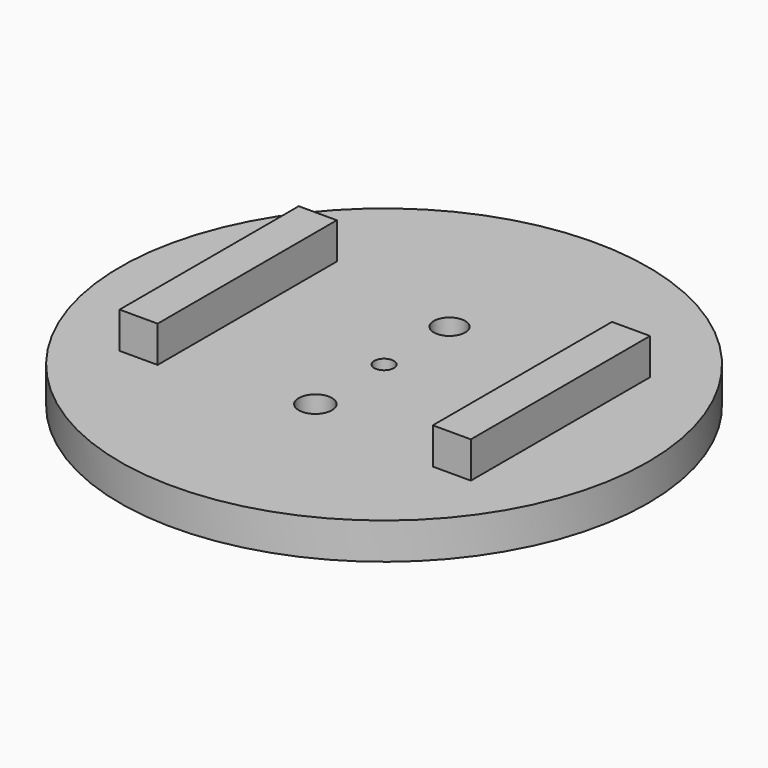
from build123d import *

# Parameters (mm, degrees)
F0_R     = 36.3144122586
F3_DEPTH = 5
F1_W     = 5.236171186
F1_H     = 30.8128492907
F4_DEPTH = 10
F2_R     = 2.2829264836
F2_R_2   = 1.3509728807
F2_R_3   = 2.1549795906
F5_DEPTH = 25
F7_DEPTH = 2


with BuildPart() as f3:
    # F0 (on Top) → F3 (new body)
    with BuildSketch(Plane.XY):
        Circle(F0_R)
    extrude(amount=F3_DEPTH)

    # F1 (on Top) → F4 (join)
    with BuildSketch(Plane.XY):
        with Locations((21.547390148, 0.1232274808)):
            Rectangle(F1_W, F1_H)
        Polygon((-24.165475741, 15.5296521261), (-24.165475741, 0), (-24.165475741, -15.2831971645), (-18.9293045551, -15.2831971645), (-18.9293045551, 15.5296521261), align=None)
    extrude(amount=F4_DEPTH)

    # F2 (on Top) → F5 (cut)
    with BuildSketch(Plane.XY):
        with Locations((0, -11.8196206167)):
            Circle(F2_R)
        Circle(F2_R_2)
        with Locations((0, 11.250000447)):
            Circle(F2_R_3)
    extrude(amount=F5_DEPTH, mode=Mode.SUBTRACT)

    # F6 (on Top) → F7 (cut)
    with BuildSketch(Plane.XY):
        with BuildLine():
            ThreePointArc((-0.3703859768, -3.5693595734), (2.402953818, -2.6652066495), (3.5885252592, 0))
            ThreePointArc((3.5885252592, 0), (2.402953818, 2.6652066495), (-0.3703859768, 3.5693595734))
            ThreePointArc((-0.3703859768, 3.5693595734), (-3.5885252592, 0), (-0.3703859768, -3.5693595734))
        make_face()
        with BuildLine():
            ThreePointArc((-0.3703859768, 3.5693595734), (2.402953818, 2.6652066495), (3.5885252592, 0))
            ThreePointArc((3.5885252592, 0), (2.402953818, -2.6652066495), (-0.3703859768, -3.5693595734))
            Line((-0.3703859768, -3.5693595734), (0, -3.6077938568))
            Line((0, -3.6077938568), (13.7103013694, -2.3183212426))
            ThreePointArc((13.7103013694, -2.3183212426), (11.3919801268, 0), (13.7103013694, 2.3183212426))
            Line((13.7103013694, 2.3183212426), (0, 3.6077938568))
            Line((0, 3.6077938568), (-0.3703859768, 3.5693595734))
        make_face()
        with BuildLine():
            ThreePointArc((-0.3703859768, -3.5693595734), (-3.5885252592, 0), (-0.3703859768, 3.5693595734))
            Line((-0.3703859768, 3.5693595734), (-12.5144906342, 2.3091877811))
            ThreePointArc((-12.5144906342, 2.3091877811), (-10.8816482952, 1.632842339), (-10.2053028531, 0))
            ThreePointArc((-10.2053028531, 0), (-10.8816482952, -1.632842339), (-12.5144906342, -2.3091877811))
            Line((-12.5144906342, -2.3091877811), (-0.3703859768, -3.5693595734))
        make_face()
        with BuildLine():
            Line((-12.5144906342, 0), (-12.5144906342, 2.3091877811))
            ThreePointArc((-12.5144906342, 2.3091877811), (-14.8236784153, 0), (-12.5144906342, -2.3091877811))
            Line((-12.5144906342, -2.3091877811), (-12.5144906342, 0))
        make_face()
        with BuildLine():
            ThreePointArc((-10.2053028531, 0), (-10.8816482952, 1.632842339), (-12.5144906342, 2.3091877811))
            Line((-12.5144906342, 2.3091877811), (-12.5144906342, 0))
            Line((-12.5144906342, 0), (-12.5144906342, -2.3091877811))
            ThreePointArc((-12.5144906342, -2.3091877811), (-10.8816482952, -1.632842339), (-10.2053028531, 0))
        make_face()
        with BuildLine():
            Line((13.7103013694, 0), (13.7103013694, 2.3183212426))
            ThreePointArc((13.7103013694, 2.3183212426), (11.3919801268, 0), (13.7103013694, -2.3183212426))
            Line((13.7103013694, -2.3183212426), (13.7103013694, 0))
        make_face()
        with BuildLine():
            ThreePointArc((16.0286226121, 0), (15.3496020411, 1.6393006716), (13.7103013694, 2.3183212426))
            Line((13.7103013694, 2.3183212426), (13.7103013694, 0))
            Line((13.7103013694, 0), (13.7103013694, -2.3183212426))
            ThreePointArc((13.7103013694, -2.3183212426), (15.3496020411, -1.6393006716), (16.0286226121, 0))
        make_face()
    extrude(amount=F7_DEPTH, mode=Mode.SUBTRACT)


solid = f3.part
